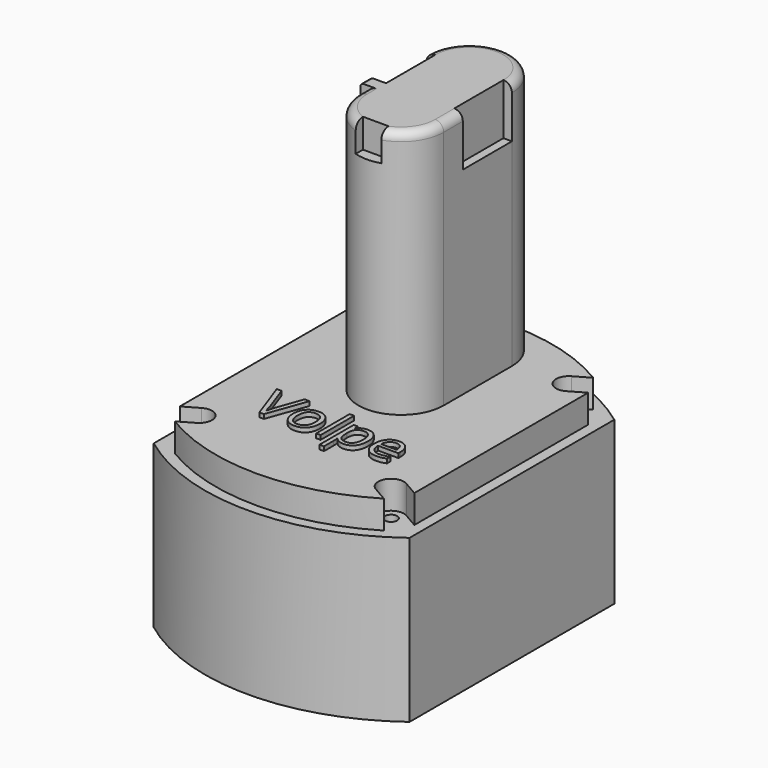
from build123d import *

# Parameters (mm, degrees)
F1_DEPTH      = 48.26
F3_DEPTH      = 8.382
F5_DEPTH      = 8.382
F6_R          = 1.8288
F7_DEPTH      = 32.8422
F9_DEPTH      = 82.55
F10_W         = 2.286
F10_H         = 3.556
F11_DEPTH     = 74.168
F12_R         = 2.54
F13_W         = 2.54
F13_H         = 18.288
F14_DEPTH     = 15.24
F16_DEPTH     = 8.636
F17_R         = 1.016
F18_TEXT_SIZE = 16.4339797468
F19_DEPTH     = 1.27


# Not quite as in the source:
# - Text() gives the source's letters only with a copy of the font that has no kerning and outlines rounded to 1/6400 em; it was checked with that copy


with BuildPart() as f1:
    # F0 (on Top) → F1 (new body)
    with BuildSketch(Plane.XY):
        with BuildLine():
            ThreePointArc((38.1, 38.1), (0, 50.8), (-38.1, 38.1))
            Line((-38.1, 38.1), (-38.1, -38.1))
            ThreePointArc((-38.1, -38.1), (0, -50.8), (38.1, -38.1))
            Line((38.1, -38.1), (38.1, 38.1))
        make_face()
    extrude(amount=-F1_DEPTH)

    # F2 (on Top) → F3 (join)
    with BuildSketch(Plane.XY):
        with BuildLine():
            Line((34.925, -36.4868884968), (34.925, 36.4868884968))
            ThreePointArc((34.925, 36.4868884968), (0, 47.625), (-34.925, 36.4868884968))
            Line((-34.925, 36.4868884968), (-34.925, -36.4868884968))
            ThreePointArc((-34.925, -36.4868884968), (0, -47.625), (34.925, -36.4868884968))
        make_face()
    extrude(amount=F3_DEPTH)

    # F4 (on face) → F5 (cut, through all)
    with BuildSketch(Plane.XY.offset(8.382)):
        with BuildLine():
            ThreePointArc((-26.67, -36.3957567884), (-25.2754432116, -31.1912), (-30.48, -29.7966432116))
            Line((-30.48, -29.7966432116), (-52.4770452561, -42.4966432116))
            ThreePointArc((-52.4770452561, -42.4966432116), (-53.8716020445, -47.7012), (-48.6670452561, -49.0957567884))
            Line((-48.6670452561, -49.0957567884), (-26.67, -36.3957567884))
        make_face()
        with BuildLine():
            ThreePointArc((30.48, -29.7966432116), (25.2754432116, -31.1912), (26.67, -36.3957567884))
            Line((26.67, -36.3957567884), (48.6670452561, -49.0957567884))
            ThreePointArc((48.6670452561, -49.0957567884), (53.8716020445, -47.7012), (52.4770452561, -42.4966432116))
            Line((52.4770452561, -42.4966432116), (30.48, -29.7966432116))
        make_face()
        with BuildLine():
            Line((-52.4770452561, 42.4966432116), (-30.48, 29.7966432116))
            ThreePointArc((-30.48, 29.7966432116), (-25.2754432116, 31.1912), (-26.67, 36.3957567884))
            Line((-26.67, 36.3957567884), (-48.6670452561, 49.0957567884))
            ThreePointArc((-48.6670452561, 49.0957567884), (-53.8716020445, 47.7012), (-52.4770452561, 42.4966432116))
        make_face()
        with BuildLine():
            Line((48.6670452561, 49.0957567884), (26.67, 36.3957567884))
            ThreePointArc((26.67, 36.3957567884), (25.2754432116, 31.1912), (30.48, 29.7966432116))
            Line((30.48, 29.7966432116), (52.4770452561, 42.4966432116))
            ThreePointArc((52.4770452561, 42.4966432116), (53.8716020445, 47.7012), (48.6670452561, 49.0957567884))
        make_face()
    extrude(amount=-F5_DEPTH, mode=Mode.SUBTRACT)

    # F6 (on face) → F7 (cut)
    with BuildSketch(Plane.XY):
        with Locations((-28.575, 33.0962)):
            Circle(F6_R)
        with Locations((28.575, 33.0962)):
            Circle(F6_R)
        with Locations((28.575, -33.0962)):
            Circle(F6_R)
        with Locations((-28.575, -33.0962)):
            Circle(F6_R)
    extrude(amount=-F7_DEPTH, mode=Mode.SUBTRACT)

    # F8 (on Top) → F9 (join)
    with BuildSketch(Plane.XY):
        with BuildLine():
            ThreePointArc((-12.7, 6.35), (0, -6.35), (12.7, 6.35))
            Line((12.7, 6.35), (12.7, 31.75))
            ThreePointArc((12.7, 31.75), (0, 44.45), (-12.7, 31.75))
            Line((-12.7, 31.75), (-12.7, 6.35))
        make_face()
    extrude(amount=F9_DEPTH)

    # F10 (on face) → F11 (join, through all)
    with BuildSketch(Plane.XY.offset(8.382)):
        with Locations((-13.843, 11.684)):
            Rectangle(F10_W, F10_H)
    extrude(amount=F11_DEPTH)

    # F12
    f12_edges = [f1.edges().sort_by_distance(p)[0] for p in [
        (12.7, 19.05, 82.55),
    ]]
    fillet(f12_edges, radius=F12_R)

    # F13 (on face) → F14 (cut)
    with BuildSketch(Plane.XY.offset(82.55)):
        with Locations((11.43, 22.606)):
            Rectangle(F13_W, F13_H)
        with Locations((-11.43, 22.606)):
            Rectangle(F13_W, F13_H)
    extrude(amount=-F14_DEPTH, mode=Mode.SUBTRACT)

    # F15 (on face) → F16 (cut)
    with BuildSketch(Plane.XY.offset(82.55)):
        with BuildLine():
            Line((3.81, -3.0685720786), (-3.81, -3.0685720786))
            Line((-3.81, -3.0685720786), (-3.81, -5.765027858))
            ThreePointArc((-3.81, -5.765027858), (0, -6.35), (3.81, -5.765027858))
            Line((3.81, -5.765027858), (3.81, -3.0685720786))
        make_face()
    extrude(amount=-F16_DEPTH, mode=Mode.SUBTRACT)

    # F17
    f17_edges = [f1.edges().sort_by_distance(p)[0] for p in [
        (-14.986, 11.684, 82.55),
    ]]
    fillet(f17_edges, radius=F17_R)

    # F18 (on face) → F19 (join)
    with BuildSketch(Plane.XY.offset(8.382)):
        with Locations((-21.2702639401, -25.0735562295)):
            Text('Volpe', F18_TEXT_SIZE, font='Open Sans', text_align=(TextAlign.LEFT, TextAlign.BOTTOM))
    extrude(amount=F19_DEPTH)


solid = f1.part
